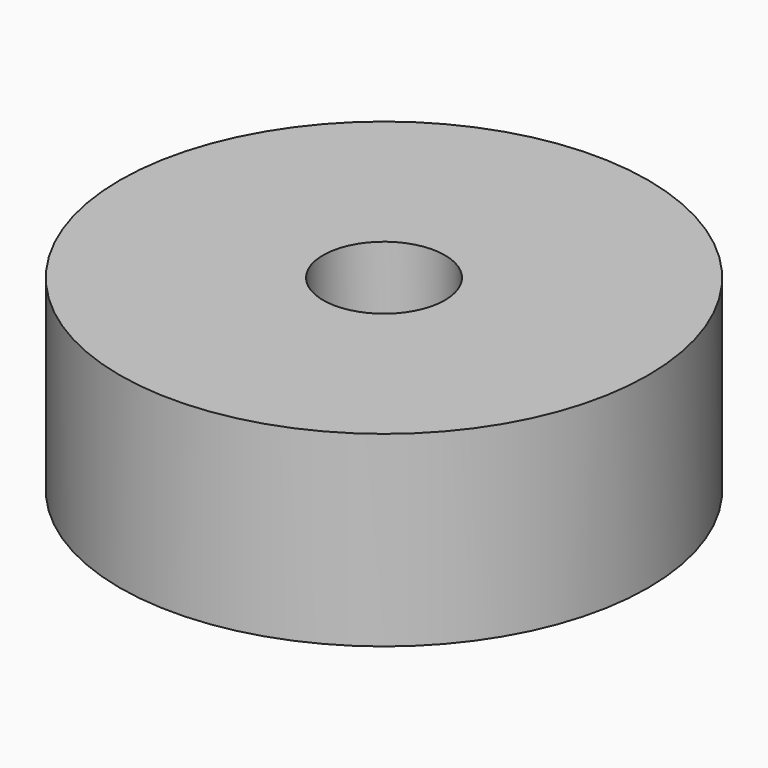
from build123d import *

# Parameters (mm, degrees)
F0_R      = 1.0216326818
F1_DEPTH  = 0.2159
F2_R      = 0.9238996
F1_FACE_R = 1.0216326818
F3_DEPTH  = 0.424434
F4_R      = 1.0216326818
F4_R_2    = 0.9238996
F5_DEPTH  = 0.508
F6_R      = 0.2356788085
F7_DEPTH  = 25.4


with BuildPart() as f1:
    # F0 (on Top) → F1 (new body)
    with BuildSketch(Plane.XY):
        Circle(F0_R)
    extrude(amount=F1_DEPTH)

    # F2 (on Top) + F1_face (on face) → F3 (cut)
    with BuildSketch(Plane.XY):
        Circle(F2_R)
    with BuildSketch(Plane.XY.offset(0.2159)):
        Circle(F1_FACE_R)
    extrude(amount=F3_DEPTH, mode=Mode.SUBTRACT)

    # F4 (on face) → F5 (join)
    with BuildSketch(Plane.XY.offset(0.2159)):
        Circle(F4_R)
        Circle(F4_R_2, mode=Mode.SUBTRACT)
        Circle(F4_R_2)
    extrude(amount=F5_DEPTH)

    # F6 (on face) → F7 (cut)
    with BuildSketch(Plane.XY.offset(0.7239)):
        Circle(F6_R)
    extrude(amount=-F7_DEPTH, mode=Mode.SUBTRACT)


solid = f1.part
